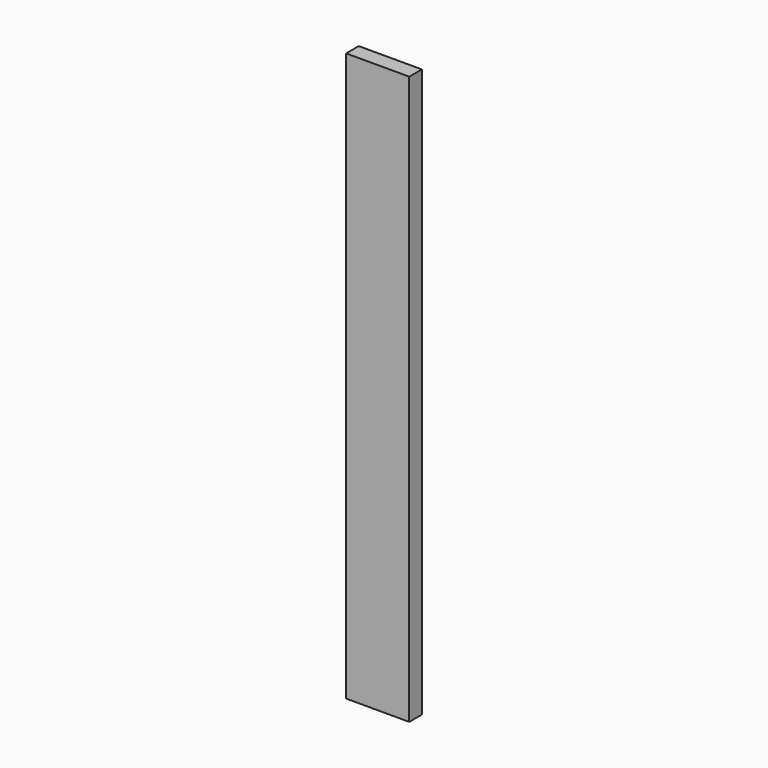
from build123d import *

# Parameters (mm, degrees)
F0_W     = 12.7
F0_H     = 114.3
F1_DEPTH = 3.175


# Not quite as in the source:
# - a length typed as a fraction of an inch, garbled in the dataset ("3 / 203.2 mm" for 3/8 in), is restored


with BuildPart() as f1:
    # F0 (on Front) → F1 (new body)
    with BuildSketch(Plane.XZ):
        with Locations((6.35, -57.15)):
            Rectangle(F0_W, F0_H)
    extrude(amount=F1_DEPTH)


solid = f1.part
